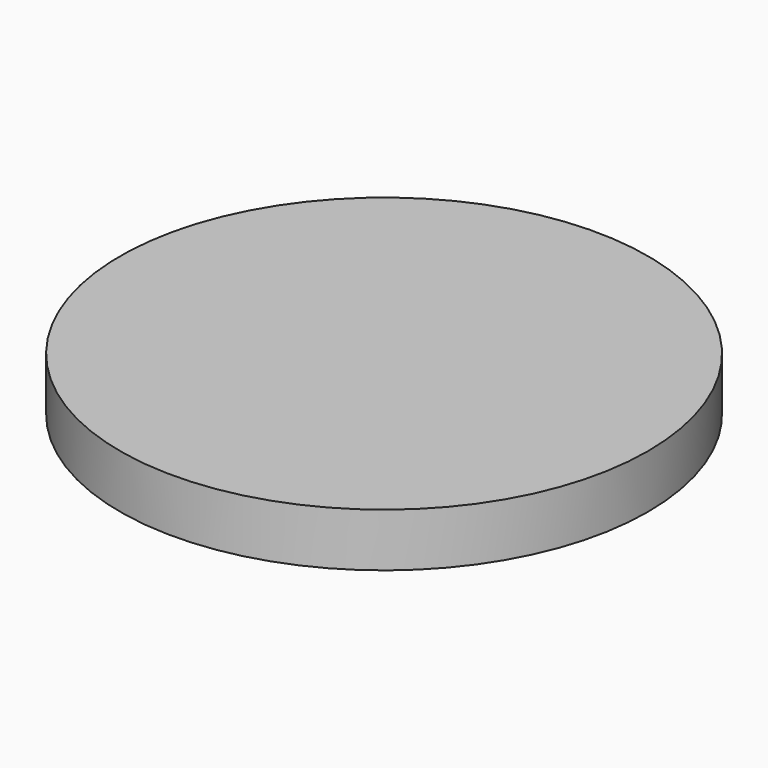
from build123d import *

# Parameters (mm, degrees)
F0_R        = 37
F0_R_2      = 35
F0_R_3      = 30
F0_R_4      = 28
F1_DEPTH    = 6
F3_R        = 3.6499996483
F6_COUNT    = 29
F8_R        = 39.5000018179
F8_R_2      = 37.5
F9_DEPTH    = 6
F8_R_3      = 27.5
F9_FACE_R   = 39.5000018179
F9_FACE_R_2 = 37.5
F9_FACE_R_3 = 27.5
F10_DEPTH   = 2


with BuildPart() as f1:
    # F0 (on Top) → F1 (new body)
    with BuildSketch(Plane.XY):
        Circle(F0_R)
        Circle(F0_R_2, mode=Mode.SUBTRACT)
        Circle(F0_R_2)
        Circle(F0_R_3, mode=Mode.SUBTRACT)
        Circle(F0_R_3)
        Circle(F0_R_4, mode=Mode.SUBTRACT)
    extrude(amount=F1_DEPTH)

    # F3 (on Front) → F4 (revolve, cut)
    with BuildSketch(Plane.XZ):
        with Locations((32.5, 3.5)):
            Circle(F3_R)
    revolve(axis=Axis((0, 0, 3.5), (0, 0, 1)), mode=Mode.SUBTRACT)


with BuildPart() as f5:
    # F2 (on Front) → F5 (revolve)
    with BuildSketch(Plane.XZ):
        with BuildLine():
            Line((32.5, 7), (32.5, 0))
            ThreePointArc((32.5, 0), (34.9748737342, 1.0251262658), (36, 3.5))
            ThreePointArc((36, 3.5), (34.9748737342, 5.9748737342), (32.5, 7))
        make_face()
    revolve(axis=Axis((32.5, 0, 3.5), (0, 0, -1)))


with BuildPart() as f6_1:
    # F6: instance of F5
    add(f5.part.rotate(Axis((0, 0, 3.5), (0, 0, 1)), 1 * 360 / F6_COUNT))


with BuildPart() as f6_2:
    # F6: instance of F5
    add(f5.part.rotate(Axis((0, 0, 3.5), (0, 0, 1)), 2 * 360 / F6_COUNT))


with BuildPart() as f6_3:
    # F6: instance of F5
    add(f5.part.rotate(Axis((0, 0, 3.5), (0, 0, 1)), 3 * 360 / F6_COUNT))


with BuildPart() as f6_4:
    # F6: instance of F5
    add(f5.part.rotate(Axis((0, 0, 3.5), (0, 0, 1)), 4 * 360 / F6_COUNT))


with BuildPart() as f6_5:
    # F6: instance of F5
    add(f5.part.rotate(Axis((0, 0, 3.5), (0, 0, 1)), 5 * 360 / F6_COUNT))


with BuildPart() as f6_6:
    # F6: instance of F5
    add(f5.part.rotate(Axis((0, 0, 3.5), (0, 0, 1)), 6 * 360 / F6_COUNT))


with BuildPart() as f6_7:
    # F6: instance of F5
    add(f5.part.rotate(Axis((0, 0, 3.5), (0, 0, 1)), 7 * 360 / F6_COUNT))


with BuildPart() as f6_8:
    # F6: instance of F5
    add(f5.part.rotate(Axis((0, 0, 3.5), (0, 0, 1)), 8 * 360 / F6_COUNT))


with BuildPart() as f6_9:
    # F6: instance of F5
    add(f5.part.rotate(Axis((0, 0, 3.5), (0, 0, 1)), 9 * 360 / F6_COUNT))


with BuildPart() as f6_10:
    # F6: instance of F5
    add(f5.part.rotate(Axis((0, 0, 3.5), (0, 0, 1)), 10 * 360 / F6_COUNT))


with BuildPart() as f6_11:
    # F6: instance of F5
    add(f5.part.rotate(Axis((0, 0, 3.5), (0, 0, 1)), 11 * 360 / F6_COUNT))


with BuildPart() as f6_12:
    # F6: instance of F5
    add(f5.part.rotate(Axis((0, 0, 3.5), (0, 0, 1)), 12 * 360 / F6_COUNT))


with BuildPart() as f6_13:
    # F6: instance of F5
    add(f5.part.rotate(Axis((0, 0, 3.5), (0, 0, 1)), 13 * 360 / F6_COUNT))


with BuildPart() as f6_14:
    # F6: instance of F5
    add(f5.part.rotate(Axis((0, 0, 3.5), (0, 0, 1)), 14 * 360 / F6_COUNT))


with BuildPart() as f6_15:
    # F6: instance of F5
    add(f5.part.rotate(Axis((0, 0, 3.5), (0, 0, 1)), 15 * 360 / F6_COUNT))


with BuildPart() as f6_16:
    # F6: instance of F5
    add(f5.part.rotate(Axis((0, 0, 3.5), (0, 0, 1)), 16 * 360 / F6_COUNT))


with BuildPart() as f6_17:
    # F6: instance of F5
    add(f5.part.rotate(Axis((0, 0, 3.5), (0, 0, 1)), 17 * 360 / F6_COUNT))


with BuildPart() as f6_18:
    # F6: instance of F5
    add(f5.part.rotate(Axis((0, 0, 3.5), (0, 0, 1)), 18 * 360 / F6_COUNT))


with BuildPart() as f6_19:
    # F6: instance of F5
    add(f5.part.rotate(Axis((0, 0, 3.5), (0, 0, 1)), 19 * 360 / F6_COUNT))


with BuildPart() as f6_20:
    # F6: instance of F5
    add(f5.part.rotate(Axis((0, 0, 3.5), (0, 0, 1)), 20 * 360 / F6_COUNT))


with BuildPart() as f6_21:
    # F6: instance of F5
    add(f5.part.rotate(Axis((0, 0, 3.5), (0, 0, 1)), 21 * 360 / F6_COUNT))


with BuildPart() as f6_22:
    # F6: instance of F5
    add(f5.part.rotate(Axis((0, 0, 3.5), (0, 0, 1)), 22 * 360 / F6_COUNT))


with BuildPart() as f6_23:
    # F6: instance of F5
    add(f5.part.rotate(Axis((0, 0, 3.5), (0, 0, 1)), 23 * 360 / F6_COUNT))


with BuildPart() as f6_24:
    # F6: instance of F5
    add(f5.part.rotate(Axis((0, 0, 3.5), (0, 0, 1)), 24 * 360 / F6_COUNT))


with BuildPart() as f6_25:
    # F6: instance of F5
    add(f5.part.rotate(Axis((0, 0, 3.5), (0, 0, 1)), 25 * 360 / F6_COUNT))


with BuildPart() as f6_26:
    # F6: instance of F5
    add(f5.part.rotate(Axis((0, 0, 3.5), (0, 0, 1)), 26 * 360 / F6_COUNT))


with BuildPart() as f6_27:
    # F6: instance of F5
    add(f5.part.rotate(Axis((0, 0, 3.5), (0, 0, 1)), 27 * 360 / F6_COUNT))


with BuildPart() as f6_28:
    # F6: instance of F5
    add(f5.part.rotate(Axis((0, 0, 3.5), (0, 0, 1)), 28 * 360 / F6_COUNT))


with BuildPart() as f9:
    # F8 (on offset) → F9 (new body)
    with BuildSketch(Plane.XY.offset(6.5)):
        Circle(F8_R)
        Circle(F8_R_2, mode=Mode.SUBTRACT)
    extrude(amount=-F9_DEPTH)



with BuildPart() as f9b:
    # F8 (on offset) → F9, piece 2 (new body)
    with BuildSketch(Plane.XY.offset(6.5)):
        Circle(F8_R_3)
    extrude(amount=-F9_DEPTH)


with BuildPart() as f9_1:
    add(f9.part)

    add(f9b.part)  # F10 merges F9b
    # F8 (on offset) + F9_face (on face) → F10 (join)
    with BuildSketch(Plane.XY.offset(6.5)):
        Circle(F8_R_2)
        Circle(F8_R_3, mode=Mode.SUBTRACT)
    with BuildSketch(Plane.XY.offset(6.5)):
        Circle(F9_FACE_R)
        Circle(F9_FACE_R_2, mode=Mode.SUBTRACT)
        Circle(F9_FACE_R_3)
    extrude(amount=F10_DEPTH)

    # F3 (on Front) → F11 (revolve, cut)
    with BuildSketch(Plane.XZ):
        with Locations((32.5, 3.5)):
            Circle(F3_R)
    revolve(axis=Axis((0, 0, 3.5), (0, 0, 1)), mode=Mode.SUBTRACT)


solid = Compound([f1.part, f5.part, f6_1.part, f6_2.part, f6_3.part, f6_4.part, f6_5.part, f6_6.part, f6_7.part, f6_8.part, f6_9.part, f6_10.part, f6_11.part, f6_12.part, f6_13.part, f6_14.part, f6_15.part, f6_16.part, f6_17.part, f6_18.part, f6_19.part, f6_20.part, f6_21.part, f6_22.part, f6_23.part, f6_24.part, f6_25.part, f6_26.part, f6_27.part, f6_28.part, f9_1.part])
